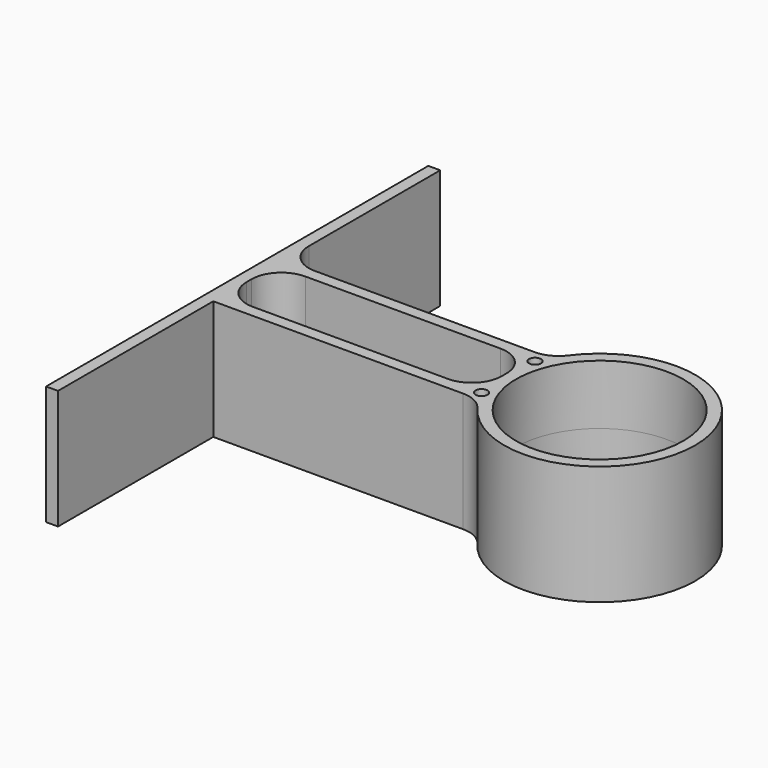
from build123d import *

# Parameters (mm, degrees)
F0_R          = 14
F1_DEPTH      = 10
F1_DEPTH_BACK = 10
F2_R          = 5
F3_R          = 5
F4_R          = 1
F5_DEPTH      = 25
F6_R          = 5


with BuildPart() as f1:
    # F0 (on Top) → F1 (new body, two sides)
    with BuildSketch(Plane.XY) as f1_sk:
        with BuildLine():
            ThreePointArc((-14.1332940251, -7.5), (3.86440782, -15.5263116097), (16, 0))
            ThreePointArc((16, 0), (3.86440782, 15.5263116097), (-14.1332940251, 7.5))
            ThreePointArc((-14.1332940251, 7.5), (-14.6133919535, 6.5152724896), (-15.0249792013, 5.5))
            ThreePointArc((-15.0249792013, 5.5), (-16, 0), (-15.0249792013, -5.5))
            ThreePointArc((-15.0249792013, -5.5), (-14.6133919535, -6.5152724896), (-14.1332940251, -7.5))
        make_face()
        Circle(F0_R, mode=Mode.SUBTRACT)
        with BuildLine():
            ThreePointArc((-15.0249792013, 5.5), (-14.6133919535, 6.5152724896), (-14.1332940251, 7.5))
            Line((-14.1332940251, 7.5), (-58.6950893998, 7.5))
            Line((-58.6950893998, 7.5), (-58.6950893998, 40))
            Line((-58.6950893998, 40), (-60.6950893998, 40))
            Line((-60.6950893998, 40), (-60.6950893998, -40))
            Line((-60.6950893998, -40), (-58.6950893998, -40))
            Line((-58.6950893998, -40), (-58.6950893998, -7.5))
            Line((-58.6950893998, -7.5), (-14.1332940251, -7.5))
            ThreePointArc((-14.1332940251, -7.5), (-14.6133919535, -6.5152724896), (-15.0249792013, -5.5))
            Line((-15.0249792013, -5.5), (-58.6950893998, -5.5))
            Line((-58.6950893998, -5.5), (-58.6950893998, 5.5))
            Line((-58.6950893998, 5.5), (-15.0249792013, 5.5))
        make_face()
    extrude(amount=F1_DEPTH)
    extrude(f1_sk.sketch, amount=-F1_DEPTH_BACK)

    # F2
    f2_edges = [f1.edges().sort_by_distance(p)[0] for p in [
        (-14.133294, -7.5, 0),
        (-15.024979, -5.5, 0),
        (-15.024979, 5.5, 0),
        (-14.133294, 7.5, 0),
    ]]
    fillet(f2_edges, radius=F2_R)

    # F3
    f3_edges = [f1.edges().sort_by_distance(p)[0] for p in [
        (-58.695089, -5.5, 0),
        (-58.695089, 5.5, 0),
    ]]
    fillet(f3_edges, radius=F3_R)

    # F4 (on face) → F5 (cut)
    with BuildSketch(Plane.XY.offset(10)):
        with Locations((-15.1501176879, -5.7808761485)):
            Circle(F4_R)
        with Locations((-15.2443397102, 5.5276307583)):
            Circle(F4_R)
    extrude(amount=-F5_DEPTH, mode=Mode.SUBTRACT)

    # F6
    f6_edges = [f1.edges().sort_by_distance(p)[0] for p in [
        (-58.695089, 7.5, 0),
    ]]
    fillet(f6_edges, radius=F6_R)


solid = f1.part
